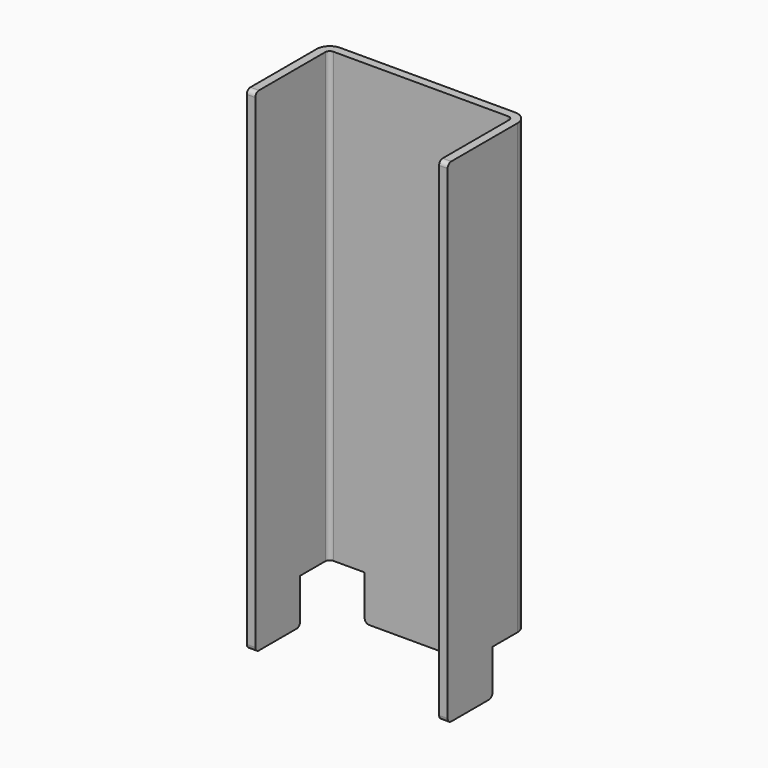
from build123d import *

# Parameters (mm, degrees)
F1_DEPTH = 50
F2_W     = 25
F2_H     = 20
F3_DEPTH = 1.9
F4_W     = 12.5
F4_H     = 10
F5_DEPTH = 1.9
F7_R     = 1


with BuildPart() as f1:
    # F0 (on Top) → F1 (new body, symmetric)
    with BuildSketch(Plane.XY):
        with BuildLine():
            Line((-19.5, 10.25), (19.5, 10.25))
            ThreePointArc((19.5, 10.25), (20.2071067812, 9.9571067812), (20.5, 9.25))
            Line((20.5, 9.25), (20.5, -10.25))
            Line((20.5, -10.25), (22.4, -10.25))
            Line((22.4, -10.25), (22.4, 9.25))
            ThreePointArc((22.4, 9.25), (21.5506096654, 11.3006096654), (19.5, 12.15))
            Line((19.5, 12.15), (-19.5, 12.15))
            ThreePointArc((-19.5, 12.15), (-21.5506096654, 11.3006096654), (-22.4, 9.25))
            Line((-22.4, 9.25), (-22.4, -10.25))
            Line((-22.4, -10.25), (-20.5, -10.25))
            Line((-20.5, -10.25), (-20.5, 9.25))
            ThreePointArc((-20.5, 9.25), (-20.2071067812, 9.9571067812), (-19.5, 10.25))
        make_face()
    extrude(amount=F1_DEPTH, both=True)

    # F2 (on face) → F3 (join, through all)
    with BuildSketch(Plane(origin=(0, 12.15, 0), x_dir=(-1, 0, 0), z_dir=(0, 1, 0))):
        with Locations((0, -50)):
            Rectangle(F2_W, F2_H)
    extrude(amount=-F3_DEPTH)

    # F4 (on face) → F5 (join, through all)
    with BuildSketch(Plane.YZ.offset(22.4)):
        with Locations((-4, -55)):
            Rectangle(F4_W, F4_H)
    extrude(amount=-F5_DEPTH)

    # F6: F1 across plane


with BuildPart() as f1_1:
    add(f1.part)
    add(f1.part.mirror(Plane.YZ))

    # F7
    f7_edges = [f1_1.edges().sort_by_distance(p)[0] for p in [
        (21.45, -10.25, 50),
        (-21.45, -10.25, 50),
        (12.5, 11.2, -60),
        (-12.5, 11.2, -60),
        (21.45, 2.25, -60),
        (-21.45, 2.25, -60),
        (21.45, -10.25, -60),
        (-21.45, -10.25, -60),
    ]]
    fillet(f7_edges, radius=F7_R)


solid = f1_1.part
